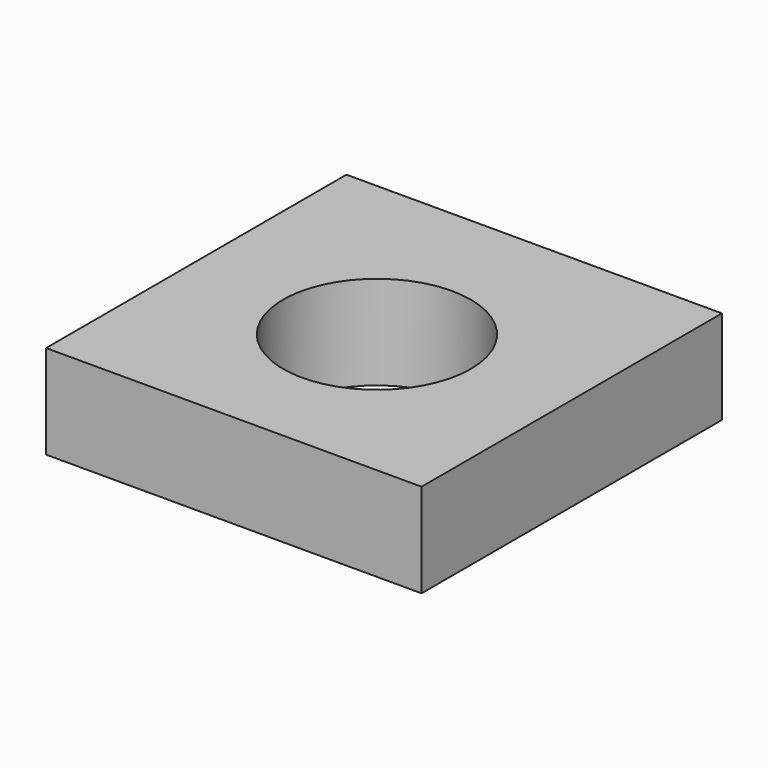
from build123d import *

# Parameters (mm, degrees)
F0_W     = 100
F0_H     = 100
F0_R     = 25
F1_DEPTH = 25


# Not quite as in the source:
# - the program builds the solid bodies; features that only make, move or delete a surface that nothing else refers to are left out


with BuildPart() as f1:
    # F0 (on Top) → F1 (new body)
    with BuildSketch(Plane.XY):
        with Locations((0.1326033846, 2.1799273789)):
            Rectangle(F0_W, F0_H)
        Circle(F0_R, mode=Mode.SUBTRACT)
    extrude(amount=F1_DEPTH)


solid = f1.part
